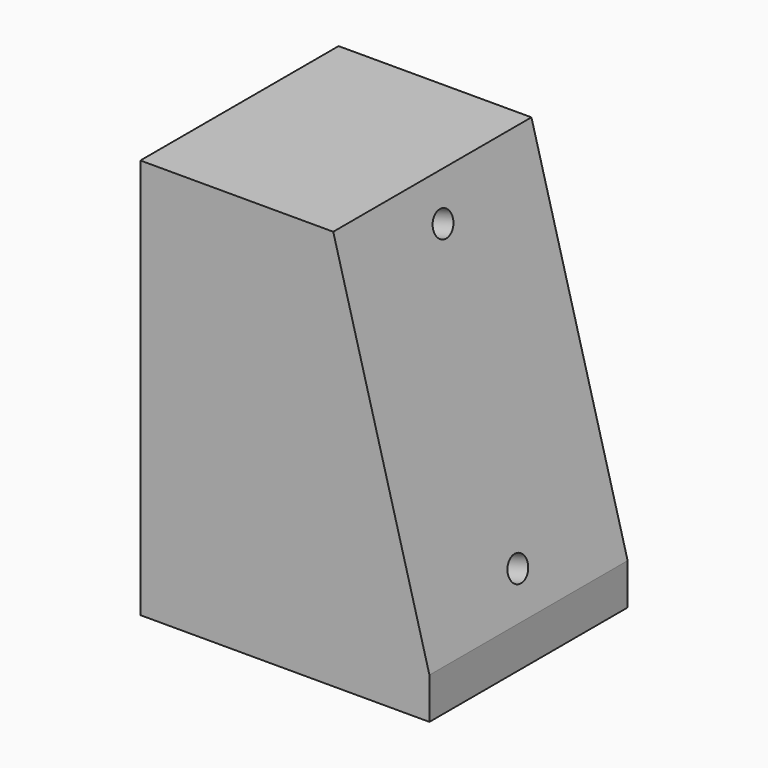
from build123d import *

# Parameters (mm, degrees)
F1_DEPTH = 60
F2_R     = 3
F3_DEPTH = 8
F4_R     = 3
F5_DEPTH = 8


# Not quite as in the source:
# - a feature names something its author has since deleted; it is built from what else it names


with BuildPart() as f1:
    # F0 (on Front) → F1 (new body)
    with BuildSketch(Plane.XZ):
        Polygon((29.4997055829, 0), (6.2059915236, 86.933324366), (-40.5002944171, 86.933324366), (-40.5002944171, -10), (29.4997055829, -10), align=None)
    extrude(amount=F1_DEPTH)

    # F2 (on face) → F3 (cut)
    with BuildSketch(Plane(origin=(0, 0, -10), x_dir=(1, 0, 0), z_dir=(0, 0, -1))):
        with Locations((-30.5002944171, 30)):
            Circle(F2_R)
        with Locations((19.4997055829, 30)):
            Circle(F2_R)
    extrude(amount=-F3_DEPTH, mode=Mode.SUBTRACT)

    # F4 (on face) → F5 (cut)
    with BuildSketch(Plane(origin=(27.5236000109, 0, 7.3749263957), x_dir=(0, 1, 0), z_dir=(0.9659258263, 0, 0.2588190451))):
        with Locations((-30, 72.3649143702)):
            Circle(F4_R)
        with Locations((-30, 2.3649143702)):
            Circle(F4_R)
    extrude(amount=-F5_DEPTH, mode=Mode.SUBTRACT)


solid = f1.part
